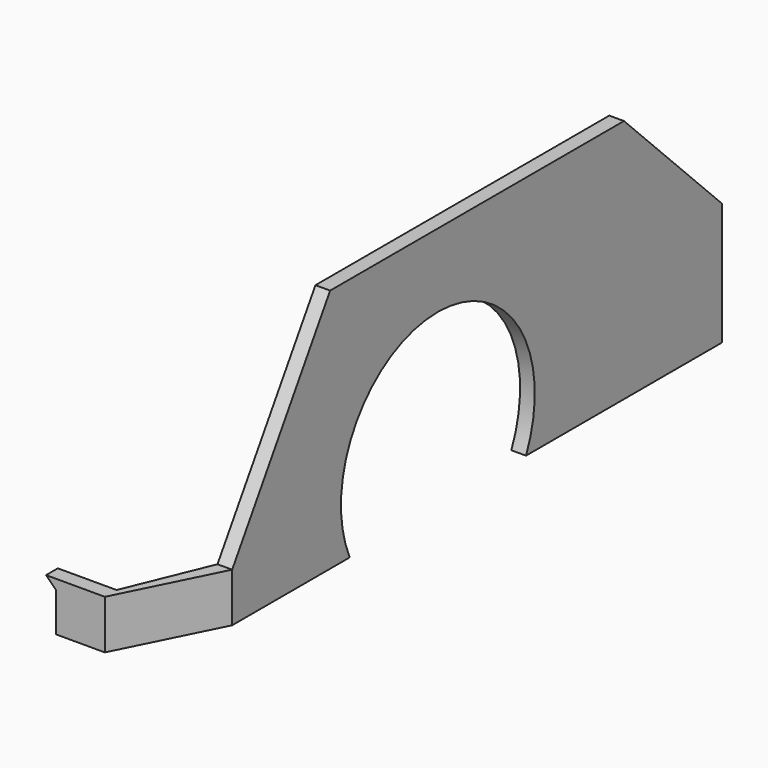
from build123d import *

# Parameters (mm, degrees)
F1_DEPTH = 10
F3_DEPTH = 3
F4_W     = 3
F4_H     = 125
F5_DEPTH = 40
F6_SIZE2 = 24.99999
F6_SIZE  = 39.99999
F7_SIZE  = 25
F9_DEPTH = 25


# Not quite as in the source:
# - a fillet or chamfer is up to 0.001 mm smaller than in the source, because OpenCascade refuses the exact size


with BuildPart() as f1:
    # F0 (on Top) → F1 (new body)
    with BuildSketch(Plane.XY):
        Polygon((0, 3), (0, 0), (10, 0), (20, 20), (20, 145), (17, 145), (17, 20), (10, 3), align=None)
    extrude(amount=F1_DEPTH)

    # F2 (on Front) → F3 (join)
    with BuildSketch(Plane.XZ):
        Polygon((0, 8), (0, 10), (-2, 10), align=None)
    extrude(amount=-F3_DEPTH)

    # F4 (on face) → F5 (join)
    with BuildSketch(Plane.XY.offset(10)):
        with Locations((18.5, 82.5)):
            Rectangle(F4_W, F4_H)
    extrude(amount=F5_DEPTH)

    # F6 (size 40 and 25 in the source; OpenCascade refuses exactly that, so slightly less here)
    f6_edges = [f1.edges().sort_by_distance(p)[0] for p in [
        (18.5, 20, 50),
    ]]
    f6_side = f1.faces().sort_by_distance((18.5, 20, 30))[0]
    chamfer(f6_edges, length=F6_SIZE, length2=F6_SIZE2, reference=f6_side)

    # F7
    f7_edges = [f1.edges().sort_by_distance(p)[0] for p in [
        (18.5, 145, 50),
    ]]
    chamfer(f7_edges, length=F7_SIZE)

    # F8 (on face) → F9 (cut)
    with BuildSketch(Plane.YZ.offset(20)):
        with BuildLine():
            Line((50, 0), (95, 0))
            ThreePointArc((95, 0), (72.5, 35), (50, 0))
        make_face()
    extrude(amount=-F9_DEPTH, mode=Mode.SUBTRACT)


solid = f1.part
